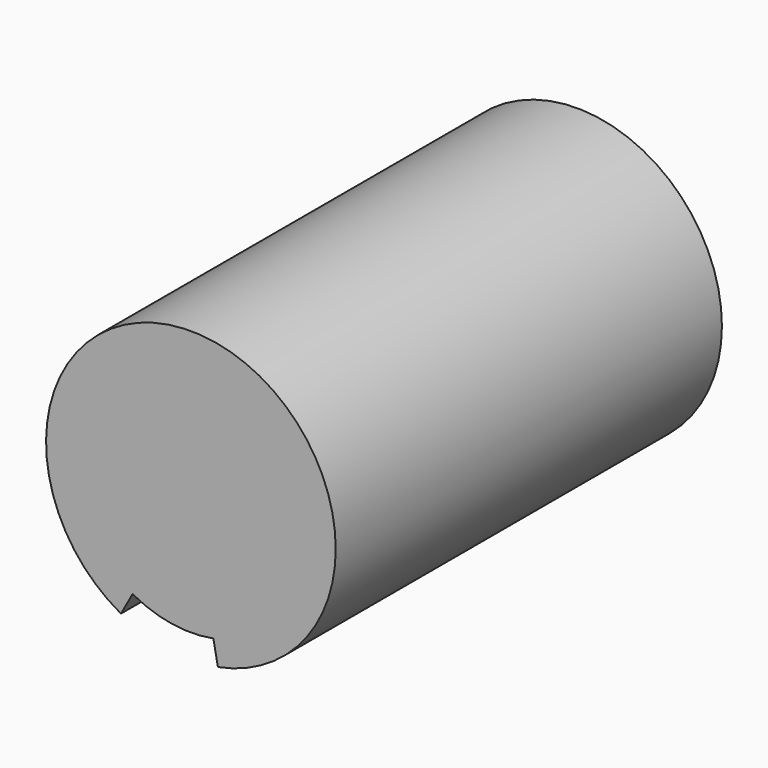
from build123d import *

# Parameters (mm, degrees)
F0_R        = 38.1
F1_DEPTH    = 127
F3_DEPTH    = 25.4
F4_T4_DEPTH = 137.1700814202
F4_S5_R     = 38.1
F4_T6_DEPTH = 76


# Not quite as in the source:
# - a fillet or chamfer that OpenCascade refuses, or shapes differently, is made with other operations: its cross-section is extruded or revolved along the edge and cut away or added


with BuildPart() as f1:
    # F0 (on Front) → F1 (new body)
    with BuildSketch(Plane.XZ):
        Circle(F0_R)
    extrude(amount=F1_DEPTH)

    # F2 (on face) → F3 (cut)
    with BuildSketch(Plane.XZ.offset(127)):
        with BuildLine():
            ThreePointArc((5.9175740903, -31.1936662944), (-5.0060402001, -31.3528636892), (-15.3369587331, -27.8000035399))
            Line((-15.3369587331, -27.8000035399), (-19.9380463531, -36.1400046019))
            ThreePointArc((-19.9380463531, -36.1400046019), (-6.5078522601, -40.758722796), (7.6928463174, -40.5517661827))
            Line((7.6928463174, -40.5517661827), (5.9175740903, -31.1936662944))
        make_face()
    extrude(amount=-F3_DEPTH, mode=Mode.SUBTRACT)

    # F4: chamfer of 25.4 x 22.86 on 1 edges, made by hand


with BuildPart() as f4_tool2:
    # F4_s3 → F4_t4 (new body)
    with BuildSketch(Plane(origin=(19.2922310235, 0, -101.6963045048), x_dir=(0, 1, 0), z_dir=(-0.1863802863, 0, 0.9824776786))):
        Polygon((-127, 0), (-101.6, 22.86), (-101.6, 0), align=None)
    extrude(amount=F4_T4_DEPTH)

    # F4_s5 → F4_t6 (intersect, symmetric)
    with BuildSketch(Plane.XZ.offset(114.3)):
        Circle(F4_S5_R)
    extrude(amount=F4_T6_DEPTH, both=True, mode=Mode.INTERSECT)

    split(bisect_by=Plane.XZ.offset(127), keep=Keep.BOTTOM)


with BuildPart() as f1_1:
    add(f1.part)

    # F4_t1: union F4_tool2
    add(f4_tool2.part)


solid = f1_1.part
